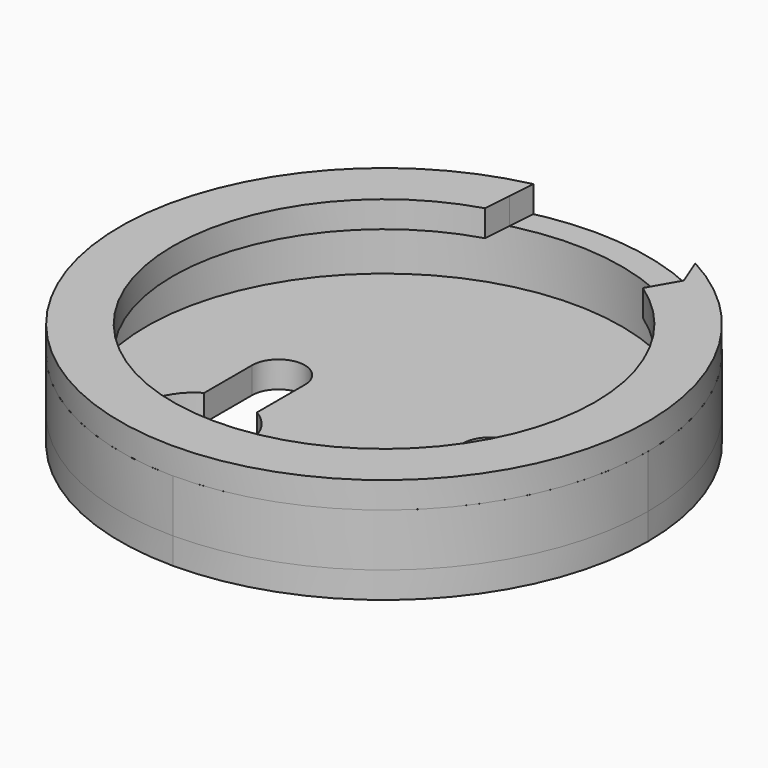
from build123d import *

# Parameters (mm, degrees)
F1_DEPTH = 5
F2_DEPTH = 10
F4_DEPTH = 5


with BuildPart() as f1:
    # F0 (on Top) → F1 (new body)
    with BuildSketch(Plane.XY):
        with BuildLine():
            ThreePointArc((0, -45), (31.8198051534, -31.8198051534), (45, 0))
            ThreePointArc((45, 0), (31.8198051534, 31.8198051534), (0, 45))
            Line((0, 45), (0, -45))
        make_face()
        with BuildLine():
            Line((15, -11.3397459622), (15, 0))
            ThreePointArc((15, 0), (20, 5), (25, 0))
            Line((25, 0), (25, -11.3397459622))
            ThreePointArc((25, -11.3397459622), (28.6602540378, -15), (30, -20))
            ThreePointArc((30, -20), (15, -28.6602540378), (15, -11.3397459622))
        make_face(mode=Mode.SUBTRACT)
        with BuildLine():
            ThreePointArc((0, 45), (31.8198051534, 31.8198051534), (45, 0))
            ThreePointArc((45, 0), (31.8198051534, -31.8198051534), (0, -45))
            Line((0, -45), (0, -50))
            ThreePointArc((0, -50), (35.3553390593, -35.3553390593), (50, 0))
            ThreePointArc((50, 0), (35.3553390593, 35.3553390593), (0, 50))
            Line((0, 50), (0, 45))
        make_face()
        with BuildLine():
            ThreePointArc((0, -45), (-45, 0), (0, 45))
            Line((0, 45), (0, 50))
            ThreePointArc((0, 50), (-50, 0), (0, -50))
            Line((0, -50), (0, -45))
        make_face()
        with BuildLine():
            Line((0, -45), (0, 45))
            ThreePointArc((0, 45), (-45, 0), (0, -45))
        make_face()
        with BuildLine():
            ThreePointArc((-25, 0), (-20, 5), (-15, 0))
            Line((-15, 0), (-15, -11.3397459622))
            ThreePointArc((-15, -11.3397459622), (-11.3397459622, -15), (-10, -20))
            ThreePointArc((-10, -20), (-25, -28.6602540378), (-25, -11.3397459622))
            Line((-25, -11.3397459622), (-25, 0))
        make_face(mode=Mode.SUBTRACT)
    extrude(amount=-F1_DEPTH)


with BuildPart() as f2:
    # F0 (on Top) → F2 (new body)
    with BuildSketch(Plane.XY):
        with BuildLine():
            ThreePointArc((0, 45), (31.8198051534, 31.8198051534), (45, 0))
            ThreePointArc((45, 0), (31.8198051534, -31.8198051534), (0, -45))
            Line((0, -45), (0, -50))
            ThreePointArc((0, -50), (35.3553390593, -35.3553390593), (50, 0))
            ThreePointArc((50, 0), (35.3553390593, 35.3553390593), (0, 50))
            Line((0, 50), (0, 45))
        make_face()
        with BuildLine():
            ThreePointArc((0, -45), (-45, 0), (0, 45))
            Line((0, 45), (0, 50))
            ThreePointArc((0, 50), (-50, 0), (0, -50))
            Line((0, -50), (0, -45))
        make_face()
    extrude(amount=F2_DEPTH)


with BuildPart() as f4:
    # F3 (on face) → F4 (new body)
    with BuildSketch(Plane.XY.offset(10)):
        with BuildLine():
            ThreePointArc((-10.7405507664, 48.8327817069), (-31.3286806432, -38.9681122093), (50, 0))
            ThreePointArc((50, 0), (42.9502428012, 25.598371888), (23.7889342673, 43.9782515162))
            Line((23.7889342673, 43.9782515162), (25.9209529209, 38.5979841529))
            Line((25.9209529209, 38.5979841529), (25.4777438216, 37.8244674206))
            Line((25.4777438216, 37.8244674206), (25.1762203925, 37.298229539))
            ThreePointArc((25.1762203925, 37.298229539), (39.7361920525, 21.1195416894), (45, 0))
            ThreePointArc((45, 0), (-27.6118154109, -35.53290939), (-11.115006654, 43.6056948928))
            Line((-11.115006654, 43.6056948928), (-10.7405507664, 48.8327817069))
        make_face()
        with BuildLine():
            Line((-11.4941642101, 38.3129767717), (-11.115006654, 43.6056948928))
            ThreePointArc((-11.115006654, 43.6056948928), (-27.6118154109, -35.53290939), (45, 0))
            ThreePointArc((45, 0), (39.7361920525, 21.1195416894), (25.1762203925, 37.298229539))
            Line((25.1762203925, 37.298229539), (22.6828947397, 32.9467188993))
            ThreePointArc((22.6828947397, 32.9467188993), (35.407031714, 18.6102688107), (40, 0))
            ThreePointArc((40, 0), (-23.8771169909, -32.0917946554), (-11.4941642101, 38.3129767717))
        make_face()
    extrude(amount=F4_DEPTH)


solid = Compound([f1.part, f2.part, f4.part])
